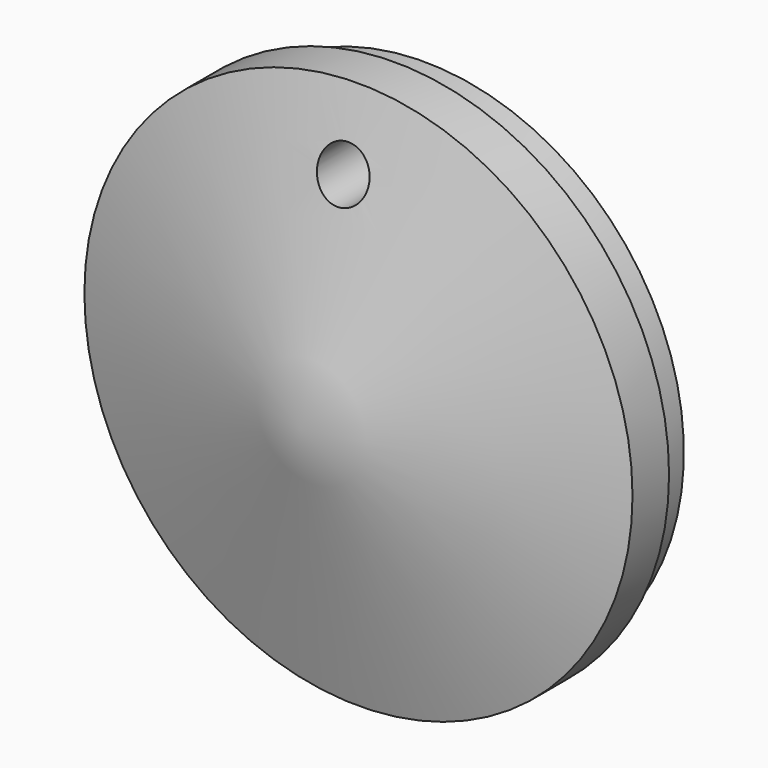
from build123d import *

# Parameters (mm, degrees)
F0_R            = 38.1
F1_DEPTH        = 6.35
F3_TEXT_SIZE    = 22.3445195136
F1_FACE1_R      = 38.1
F4_DEPTH        = 5.08
F6_R            = 3.5813937616
F7_DEPTH        = 25.4
F8_DEPTH        = 5.08
F9_R            = 36.0966045799
F9_R_2          = 31.9190281221
F10_DEPTH       = 5.08
F2_TEXT_SIZE    = 41.4397127719
F11_DEPTH       = 5.08
F12_TEXT_SIZE   = 6.4763495922
F12_TEXT_SIZE_2 = 7.1744378691
F14_DEPTH       = 5.08
F13_TEXT_SIZE   = 7.5802569174
F15_DEPTH       = 5.08


# Not quite as in the source:
# - an extrude whose draft closes it to a point is written as a loft to that point
# - Text() gives the source's letters only with a copy of the font that has no kerning and outlines rounded to 1/6400 em; it was checked with that copy


with BuildPart() as f1:
    # F0 (on Front) → F1 (new body)
    with BuildSketch(Plane.XZ):
        Circle(F0_R)
    extrude(amount=-F1_DEPTH)

    # F3 (on face) + F1_face1 (on face) → F4 (cut)
    with BuildSketch(Plane(origin=(0, 6.35, 0), x_dir=(-1, 0, 0), z_dir=(0, 1, 0))):
        with Locations((-12.2819624958, -3.3240339544)):
            Text('ubs', F3_TEXT_SIZE, font='Open Sans', font_style=FontStyle.BOLD, text_align=(TextAlign.LEFT, TextAlign.BOTTOM))
    with BuildSketch(Plane.XZ):
        Circle(F1_FACE1_R)
    extrude(amount=-F4_DEPTH, dir=(0, 1, 0), mode=Mode.SUBTRACT)

    # F1_face1 (on face) → F5 section 0
    with BuildSketch(Plane.XZ, mode=Mode.PRIVATE) as f5_s0:
        Circle(F1_FACE1_R)
    loft([f5_s0.sketch, Vertex(0, -10.2088642316, 0)], ruled=True)

    # F6 (on face) → F7 (cut)
    with BuildSketch(Plane(origin=(0, 6.35, 0), x_dir=(-1, 0, 0), z_dir=(0, 1, 0))):
        with Locations((0, 28.0307866633)):
            Circle(F6_R)
    extrude(amount=-F7_DEPTH, mode=Mode.SUBTRACT)

    # F8 (cut): faces of the model
    f8_faces = [f1.faces().sort_by_distance(p)[0] for p in [
        (7.4430243051, 1.27, 5.3117737045),
        (-15.3340137737, 1.27, 2.8606640601),
        (-22.1187719476, 1.27, 2.7370323686),
    ]]
    extrude(f8_faces, amount=F8_DEPTH, mode=Mode.SUBTRACT)

    # F9 (on face) → F10 (join)
    with BuildSketch(Plane(origin=(0, 6.35, 0), x_dir=(-1, 0, 0), z_dir=(0, 1, 0))):
        Circle(F9_R)
        Circle(F9_R_2, mode=Mode.SUBTRACT)
    extrude(amount=F10_DEPTH)

    # F2 (on face) → F11 (join)
    with BuildSketch(Plane(origin=(0, 6.35, 0), x_dir=(-1, 0, 0), z_dir=(0, 1, 0))):
        with Locations((-31.8915654934, -11.8254980023)):
            Text('C', F2_TEXT_SIZE, font='Open Sans', font_style=FontStyle.BOLD, text_align=(TextAlign.LEFT, TextAlign.BOTTOM))
    extrude(amount=F11_DEPTH)

    # F12 (on face) → F14 (cut)
    with BuildSketch(Plane(origin=(0, 6.35, 0), x_dir=(-1, 0, 0), z_dir=(0, 1, 0))):
        with Locations((0, -11.5056402422)):
            Text('2016', F12_TEXT_SIZE, font='Open Sans', font_style=FontStyle.BOLD, text_align=(TextAlign.LEFT, TextAlign.BOTTOM))
        with Locations((-22.432449406, -18.0551351935)):
            Text('World Series', F12_TEXT_SIZE_2, font='Open Sans', font_style=FontStyle.BOLD, text_align=(TextAlign.LEFT, TextAlign.BOTTOM))
    extrude(amount=-F14_DEPTH, mode=Mode.SUBTRACT)

    # F13 (on face) → F15 (cut)
    with BuildSketch(Plane(origin=(0, 6.35, 0), x_dir=(-1, 0, 0), z_dir=(0, 1, 0))):
        with Locations((-21.7083727475, -24.361345917)):
            Text('Champions', F13_TEXT_SIZE, font='Open Sans', font_style=FontStyle.BOLD, text_align=(TextAlign.LEFT, TextAlign.BOTTOM))
    extrude(amount=-F15_DEPTH, mode=Mode.SUBTRACT)


solid = f1.part
